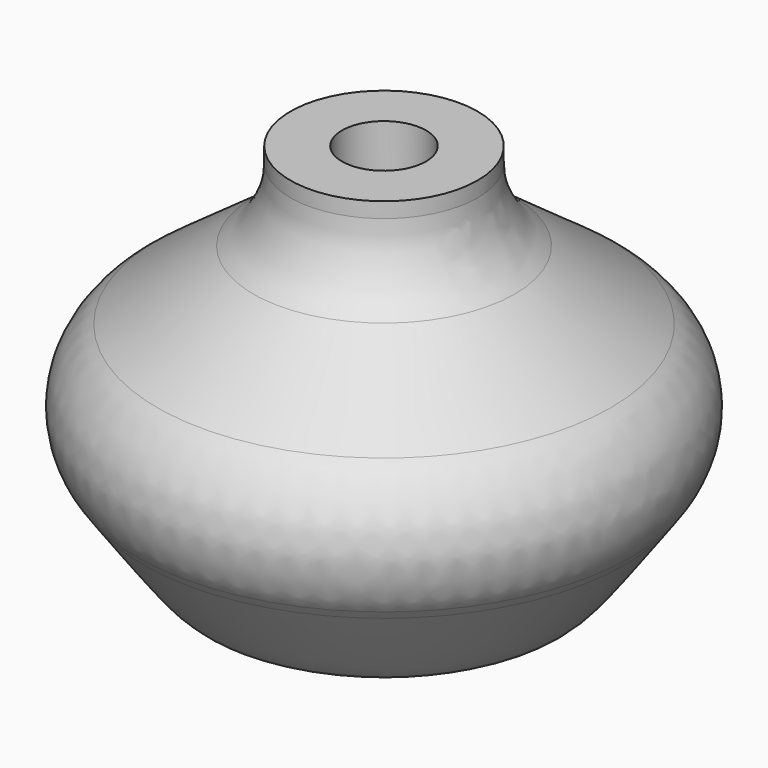
from build123d import *

# Parameters (mm, degrees)
F2_R     = 10.16
F3_R     = 10.16
F5_R     = 4.7752
F6_DEPTH = 10.795
F7_R     = 1.59385
F8_DEPTH = 20.32


# Not quite as in the source:
# - a fillet or chamfer that OpenCascade refuses, or shapes differently, is made with other operations: its cross-section is extruded or revolved along the edge and cut away or added


with BuildPart() as f1:
    # F0 (on Front) → F1 (revolve)
    with BuildSketch(Plane.XZ):
        Polygon((0, 50.8), (0, 0), (6.8085049027, 15.3191369531), (19.1836198036, 6.4245244719), (34.007973939, 27.0497159733), (10.633115835, 43.8503926785), (10.633115835, 50.8), align=None)
    revolve(axis=Axis((0, 0, 25.4), (0, 0, -1)))

    # F2
    f2_edges = [f1.edges().sort_by_distance(p)[0] for p in [
        (-10.633116, 0, 43.850393),
    ]]
    fillet(f2_edges, radius=F2_R)

    # F3
    f3_edges = [f1.edges().sort_by_distance(p)[0] for p in [
        (24.435674, 0, 33.929805),
        (-14.86337, 0, 40.809895),
        (-34.007974, 0, 27.049716),
    ]]
    fillet(f3_edges, radius=F3_R)

    # F4: fillet of radius 13.97 on 3 edges, made by hand

    # F4_s1 → F4_t2 (revolve, cut)
    with BuildSketch(Plane.XZ):
        with BuildLine():
            add(Edge.make_bspline(
                [(27.337014578, 17.7683797976), (19.1836198036, 6.4245244719), (7.8397644778, 14.5779192464)],
                knots=[0, 0, 0, 1, 1, 1], degree=2, weights=[1, 7.3333333333, 1]))
            Line((7.8397644778, 14.5779192464), (19.1836198036, 6.4245244719))
            Line((19.1836198036, 6.4245244719), (27.337014578, 17.7683797976))
        make_face()
    revolve(axis=Axis((0, 0, 6.4245244719), (0, 0, -1)), mode=Mode.SUBTRACT)

    # F5 (on face) → F6 (cut)
    with BuildSketch(Plane.XY.offset(50.8)):
        Circle(F5_R)
    extrude(amount=-F6_DEPTH, mode=Mode.SUBTRACT)

    # F7 (on Top) → F8 (cut)
    with BuildSketch(Plane.XY):
        Circle(F7_R)
    extrude(amount=F8_DEPTH, mode=Mode.SUBTRACT)


solid = f1.part
